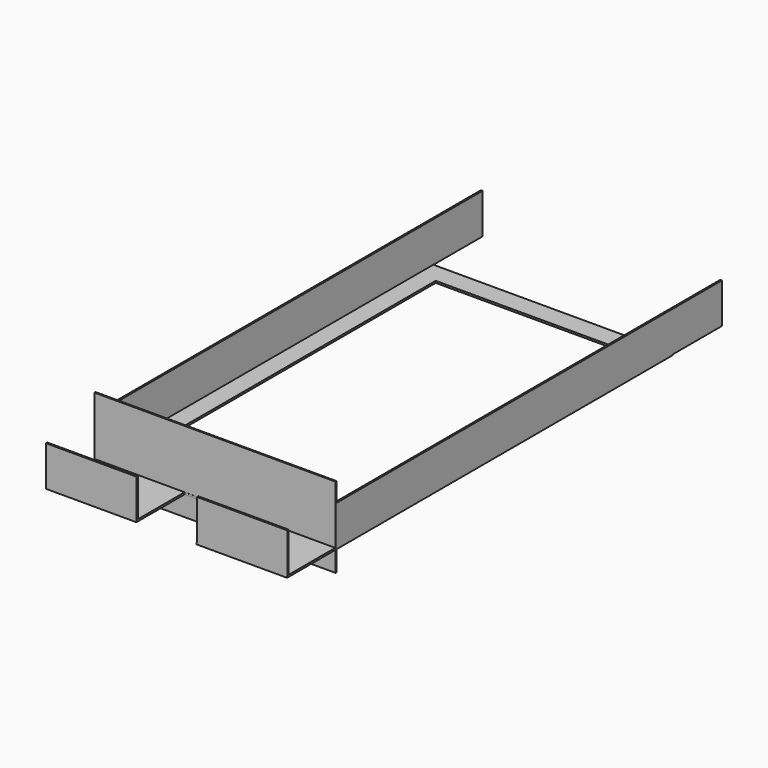
from build123d import *

# Parameters (mm, degrees)
F0_W      = 1219.2
F0_H      = 2438.4
F0_W_2    = 1016
F0_H_2    = 2032
F1_DEPTH  = 9.525
F2_DEPTH  = 9.525
F4_START  = 908.05
F3_W      = 1219.2
F3_H      = 406.4
F4_DEPTH  = 6.35
F6_START  = 601.345
F5_W      = 2438.4
F5_H      = 203.2
F6_DEPTH  = 8.255
F8_START  = -601.345
F7_W      = 2438.4
F7_H      = 203.2
F8_DEPTH  = 8.255
F10_W     = 304.8
F10_H     = 304.8
F11_DEPTH = 43.18
F12_START = 1210.945
F9_W      = 457.2
F9_H      = 203.2
F12_DEPTH = 8.255
F14_START = 1210.945
F13_W     = 457.2
F13_H     = 203.2
F14_DEPTH = 8.255


# Not quite as in the source:
# - a feature names something its author has since deleted; it is built from what else it names


with BuildPart() as f1:
    # F0 (on Top) → F1 (new body)
    with BuildSketch(Plane.XY):
        Rectangle(F0_W, F0_H)
        with Locations((0, 101.6)):
            Rectangle(F0_W_2, F0_H_2, mode=Mode.SUBTRACT)
    extrude(amount=F1_DEPTH)

    # F0 (on Top) → F2 (cut)
    with BuildSketch(Plane.XY):
        Rectangle(F0_W, F0_H)
        with Locations((0, 101.6)):
            Rectangle(F0_W_2, F0_H_2, mode=Mode.SUBTRACT)
    extrude(amount=-F2_DEPTH, mode=Mode.SUBTRACT)

    # F3 (on Front) → F4 (join)
    with BuildSketch(Plane.XZ.offset(F4_START)):
        with Locations((1.2260880321, 101.6)):
            Rectangle(F3_W, F3_H)
    extrude(amount=F4_DEPTH)

    # F5 (on Right) → F6 (join)
    with BuildSketch(Plane.YZ.offset(F6_START)):
        with Locations((311.4953897893, 105.20761006)):
            Rectangle(F5_W, F5_H)
    extrude(amount=F6_DEPTH)

    # F7 (on Right) → F8 (join)
    with BuildSketch(Plane.YZ.offset(F8_START)):
        with Locations((311.7190003395, 110.4580410756)):
            Rectangle(F7_W, F7_H)
    extrude(amount=-F8_DEPTH)

    # F10 (on Top) → F11 (cut)
    with BuildSketch(Plane.XY):
        with Locations((0, -1067.1225335449)):
            Rectangle(F10_W, F10_H)
    extrude(amount=F11_DEPTH, mode=Mode.SUBTRACT)

    # F9 (on Front) → F12 (join)
    with BuildSketch(Plane.XZ.offset(F12_START)):
        with Locations((-381.010832265, 101.2114638133)):
            Rectangle(F9_W, F9_H)
    extrude(amount=F12_DEPTH)

    # F13 (on Front) → F14 (join)
    with BuildSketch(Plane.XZ.offset(F14_START)):
        with Locations((382.1813091636, 110.2889241311)):
            Rectangle(F13_W, F13_H)
    extrude(amount=F14_DEPTH)


solid = f1.part
